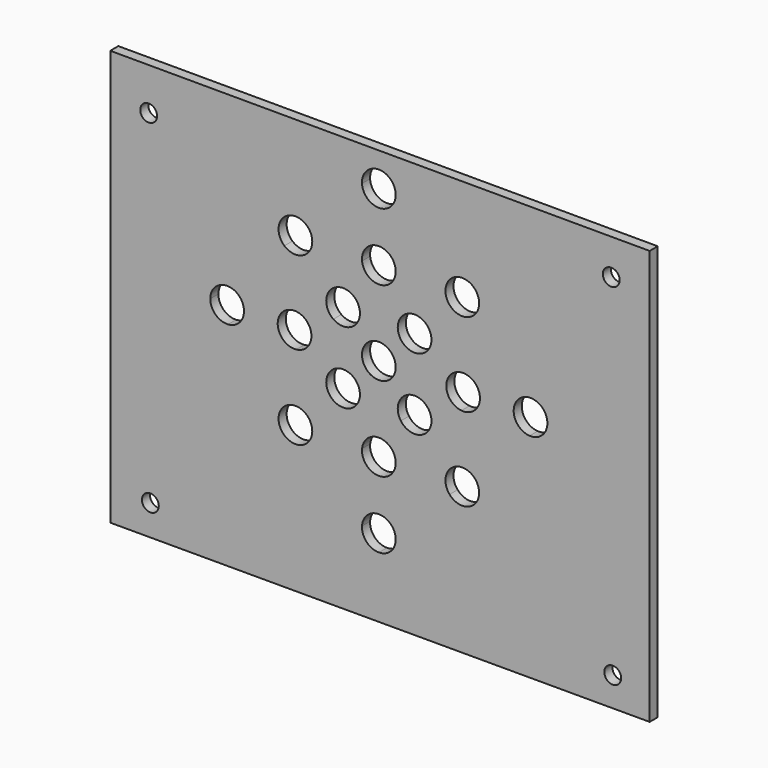
from build123d import *

# Parameters (mm, degrees)
F0_R     = 2.5
F0_R_2   = 5
F1_DEPTH = 3


with BuildPart() as f1:
    # F0 (on Front) → F1 (new body)
    with BuildSketch(Plane.XZ):
        Polygon((0, -68), (80, -68), (80, 55), (-80, 55.240198642), (-80, -68), align=None)
        with Locations((-68.1081116199, -58.9685998857)):
            Circle(F0_R, mode=Mode.SUBTRACT)
        with Locations((69.0506994724, -59.3423657119)):
            Circle(F0_R, mode=Mode.SUBTRACT)
        Polygon((49.6701618657, 0.1303526806), (49.6701618657, -49.8696473194), (-0.3298381532, -49.8696473194), (-50.3298381343, -49.8696473194), (-50.3298381343, 0.130352625), (-50.3298381343, 50.1303526806), (-0.3298380849, 50.1303526806), (49.6701618657, 50.1303526806), align=None, mode=Mode.SUBTRACT)
        with Locations((-68.6089098454, 42.6927655935)):
            Circle(F0_R, mode=Mode.SUBTRACT)
        with Locations((68.6089023948, 44.4455519319)):
            Circle(F0_R, mode=Mode.SUBTRACT)
        with BuildLine():
            ThreePointArc((-45.0520603566, -4.8619253071), (-32.1496432877, -31.6894524728), (-5.322116122, -44.5918695417))
            ThreePointArc((-5.322116122, -44.5918695417), (-0.3298381343, -39.8696473194), (4.6624398533, -44.5918695417))
            ThreePointArc((4.6624398533, -44.5918695417), (31.489967019, -31.6894524728), (44.3923840879, -4.8619253071))
            ThreePointArc((44.3923840879, -4.8619253071), (39.6701618657, 0.1303526806), (44.3923840879, 5.1226306682))
            ThreePointArc((44.3923840879, 5.1226306682), (31.489967019, 31.950157834), (4.6624398533, 44.8525749028))
            ThreePointArc((4.6624398533, 44.8525749028), (-0.3298381343, 40.1303526806), (-5.322116122, 44.8525749028))
            ThreePointArc((-5.322116122, 44.8525749028), (-32.1496432877, 31.950157834), (-45.0520603566, 5.1226306682))
            ThreePointArc((-45.0520603566, 5.1226306682), (-41.6974223481, 3.5662740353), (-40.3298381343, 0.1303526806))
            ThreePointArc((-40.3298381343, 0.1303526806), (-41.6974223481, -3.3055686741), (-45.0520603566, -4.8619253071))
        make_face()
        with BuildLine():
            ThreePointArc((27.6928642243, 21.1000487327), (32.8800593553, 11.1803621251), (34.6701618657, 0.1303526806))
            ThreePointArc((34.6701618657, 0.1303526806), (32.8800593553, -10.9196567639), (27.6928642243, -20.8393433716))
            ThreePointArc((27.6928642243, -20.8393433716), (28.9669661089, -22.5411058021), (29.4188992072, -24.618384661))
            ThreePointArc((29.4188992072, -24.618384661), (26.1660101872, -29.303211576), (20.6398579178, -27.8923496781))
            ThreePointArc((20.6398579178, -27.8923496781), (-0.3298381343, -34.8696473194), (-21.2995341865, -27.8923496781))
            ThreePointArc((-21.2995341865, -27.8923496781), (-28.6141093818, -28.1539185669), (-28.352540493, -20.8393433716))
            ThreePointArc((-28.352540493, -20.8393433716), (-35.3298381343, 0.1303526806), (-28.352540493, 21.1000487327))
            ThreePointArc((-28.352540493, 21.1000487327), (-28.6141093818, 28.414623928), (-21.2995341865, 28.1530550392))
            ThreePointArc((-21.2995341865, 28.1530550392), (-0.3298381343, 35.1303526806), (20.6398579178, 28.1530550392))
            ThreePointArc((20.6398579178, 28.1530550392), (26.1660101872, 29.5639169371), (29.4188992072, 24.8790900221))
            ThreePointArc((29.4188992072, 24.8790900221), (28.9669661089, 22.8018111633), (27.6928642243, 21.1000487327))
        make_face(mode=Mode.SUBTRACT)
        with BuildLine():
            ThreePointArc((27.6928642243, -20.8393433716), (32.8800593553, -10.9196567639), (34.6701618657, 0.1303526806))
            ThreePointArc((34.6701618657, 0.1303526806), (32.8800593553, 11.1803621251), (27.6928642243, 21.1000487327))
            ThreePointArc((27.6928642243, 21.1000487327), (20.8833653012, 21.3435561162), (20.6398579178, 28.1530550392))
            ThreePointArc((20.6398579178, 28.1530550392), (-0.3298381343, 35.1303526806), (-21.2995341865, 28.1530550392))
            ThreePointArc((-21.2995341865, 28.1530550392), (-20.3937485609, 26.6262010021), (-20.0785754759, 24.8790900221))
            ThreePointArc((-20.0785754759, 24.8790900221), (-23.0012966171, 20.3310231204), (-28.352540493, 21.1000487327))
            ThreePointArc((-28.352540493, 21.1000487327), (-35.3298381343, 0.1303526806), (-28.352540493, -20.8393433716))
            ThreePointArc((-28.352540493, -20.8393433716), (-23.0012966171, -20.0703177592), (-20.0785754759, -24.618384661))
            ThreePointArc((-20.0785754759, -24.618384661), (-20.3937485609, -26.365495641), (-21.2995341865, -27.8923496781))
            ThreePointArc((-21.2995341865, -27.8923496781), (-0.3298381343, -34.8696473194), (20.6398579178, -27.8923496781))
            ThreePointArc((20.6398579178, -27.8923496781), (20.8833653012, -21.082850755), (27.6928642243, -20.8393433716))
        make_face()
        with BuildLine():
            ThreePointArc((4.6450990512, 24.6303526806), (17.3478313953, 17.8080222102), (24.1701618657, 5.1052898661))
            ThreePointArc((24.1701618657, 5.1052898661), (28.0242638319, 3.8384519241), (29.6701618657, 0.1303526806))
            ThreePointArc((29.6701618657, 0.1303526806), (28.0242638319, -3.577746563), (24.1701618657, -4.844584505))
            ThreePointArc((24.1701618657, -4.844584505), (17.3478313953, -17.5473168491), (4.6450990512, -24.3696473194))
            ThreePointArc((4.6450990512, -24.3696473194), (4.6638922312, -24.6193334441), (4.6701618657, -24.8696473194))
            ThreePointArc((4.6701618657, -24.8696473194), (-0.5801520096, -29.863377685), (-5.3047753199, -24.3696473194))
            ThreePointArc((-5.3047753199, -24.3696473194), (-18.007507664, -17.5473168491), (-24.8298381343, -4.844584505))
            ThreePointArc((-24.8298381343, -4.844584505), (-30.3298381343, 0.1303526806), (-24.8298381343, 5.1052898661))
            ThreePointArc((-24.8298381343, 5.1052898661), (-18.007507664, 17.8080222102), (-5.3047753199, 24.6303526806))
            ThreePointArc((-5.3047753199, 24.6303526806), (-0.5801520096, 30.1240830461), (4.6701618657, 25.1303526806))
            ThreePointArc((4.6701618657, 25.1303526806), (4.6638922312, 24.8800388053), (4.6450990512, 24.6303526806))
        make_face(mode=Mode.SUBTRACT)
        with BuildLine():
            ThreePointArc((24.1701618657, -4.844584505), (19.6701618657, 0.1303526806), (24.1701618657, 5.1052898661))
            ThreePointArc((24.1701618657, 5.1052898661), (17.3478313953, 17.8080222102), (4.6450990512, 24.6303526806))
            ThreePointArc((4.6450990512, 24.6303526806), (-0.3298381343, 20.1303526806), (-5.3047753199, 24.6303526806))
            ThreePointArc((-5.3047753199, 24.6303526806), (-18.007507664, 17.8080222102), (-24.8298381343, 5.1052898661))
            ThreePointArc((-24.8298381343, 5.1052898661), (-21.6217388908, 3.4844546468), (-20.3298381343, 0.1303526806))
            ThreePointArc((-20.3298381343, 0.1303526806), (-21.6217388908, -3.2237492857), (-24.8298381343, -4.844584505))
            ThreePointArc((-24.8298381343, -4.844584505), (-18.007507664, -17.5473168491), (-5.3047753199, -24.3696473194))
            ThreePointArc((-5.3047753199, -24.3696473194), (-0.3298381343, -19.8696473194), (4.6450990512, -24.3696473194))
            ThreePointArc((4.6450990512, -24.3696473194), (17.3478313953, -17.5473168491), (24.1701618657, -4.844584505))
        make_face()
        with BuildLine():
            ThreePointArc((13.1735913764, 6.6616153035), (14.2912330073, 3.4806181431), (14.6701618657, 0.1303526806))
            ThreePointArc((14.6701618657, 0.1303526806), (14.2912330073, -3.219912782), (13.1735913764, -6.4009099423))
            ThreePointArc((13.1735913764, -6.4009099423), (14.7199684496, -8.1832312619), (15.2767635834, -10.4762490372))
            ThreePointArc((15.2767635834, -10.4762490372), (11.7971754562, -15.2394777465), (6.2014244886, -13.3730768301))
            ThreePointArc((6.2014244886, -13.3730768301), (-0.3298381343, -14.8696473194), (-6.8611007573, -13.3730768301))
            ThreePointArc((-6.8611007573, -13.3730768301), (-14.4719737581, -14.0117829432), (-13.833267645, -6.4009099423))
            ThreePointArc((-13.833267645, -6.4009099423), (-15.3298381343, 0.1303526806), (-13.833267645, 6.6616153035))
            ThreePointArc((-13.833267645, 6.6616153035), (-14.4719737581, 14.2724883043), (-6.8611007573, 13.6337821913))
            ThreePointArc((-6.8611007573, 13.6337821913), (-0.3298381343, 15.1303526806), (6.2014244886, 13.6337821913))
            ThreePointArc((6.2014244886, 13.6337821913), (11.7971754562, 15.5001831077), (15.2767635834, 10.7369543984))
            ThreePointArc((15.2767635834, 10.7369543984), (14.7199684496, 8.4439366231), (13.1735913764, 6.6616153035))
        make_face(mode=Mode.SUBTRACT)
        with BuildLine():
            Line((-0.3298381532, -49.8696473194), (49.6701618657, -49.8696473194))
            Line((49.6701618657, -49.8696473194), (49.6701618657, 0.1303526806))
            ThreePointArc((49.6701618657, 0.1303526806), (48.1060832203, -3.5020631057), (44.3923840879, -4.8619253071))
            ThreePointArc((44.3923840879, -4.8619253071), (31.489967019, -31.6894524728), (4.6624398533, -44.5918695417))
            ThreePointArc((4.6624398533, -44.5918695417), (4.6682309897, -44.7307047744), (4.6701618657, -44.8696473194))
            ThreePointArc((4.6701618657, -44.8696473194), (3.2056957649, -48.405181232), (-0.3298381532, -49.8696473194))
        make_face()
        with BuildLine():
            Line((-50.3298381343, -49.8696473194), (-0.3298381532, -49.8696473194))
            ThreePointArc((-0.3298381532, -49.8696473194), (-3.9622539271, -48.3055686673), (-5.322116122, -44.5918695417))
            ThreePointArc((-5.322116122, -44.5918695417), (-32.1496432877, -31.6894524728), (-45.0520603566, -4.8619253071))
            ThreePointArc((-45.0520603566, -4.8619253071), (-48.7657594688, -3.5020631248), (-50.3298381343, 0.130352625))
            Line((-50.3298381343, 0.130352625), (-50.3298381343, -49.8696473194))
        make_face()
        with BuildLine():
            ThreePointArc((44.3923840879, 5.1226306682), (48.1060832203, 3.7627684669), (49.6701618657, 0.1303526806))
            Line((49.6701618657, 0.1303526806), (49.6701618657, 50.1303526806))
            Line((49.6701618657, 50.1303526806), (-0.3298380849, 50.1303526806))
            ThreePointArc((-0.3298380849, 50.1303526806), (3.205695789, 48.665886569), (4.6701618657, 45.1303526806))
            ThreePointArc((4.6701618657, 45.1303526806), (4.6682309897, 44.9914101355), (4.6624398533, 44.8525749028))
            ThreePointArc((4.6624398533, 44.8525749028), (31.489967019, 31.950157834), (44.3923840879, 5.1226306682))
        make_face()
        with BuildLine():
            Line((-50.3298381343, 50.1303526806), (-50.3298381343, 0.130352625))
            ThreePointArc((-50.3298381343, 0.130352625), (-48.7657595092, 3.7627684478), (-45.0520603566, 5.1226306682))
            ThreePointArc((-45.0520603566, 5.1226306682), (-32.1496432877, 31.950157834), (-5.322116122, 44.8525749028))
            ThreePointArc((-5.322116122, 44.8525749028), (-3.9622539037, 48.5662740532), (-0.3298380849, 50.1303526806))
            Line((-0.3298380849, 50.1303526806), (-50.3298381343, 50.1303526806))
        make_face()
        with BuildLine():
            ThreePointArc((13.1735913764, -6.4009099423), (14.2912330073, -3.219912782), (14.6701618657, 0.1303526806))
            ThreePointArc((14.6701618657, 0.1303526806), (14.2912330073, 3.4806181431), (13.1735913764, 6.6616153035))
            ThreePointArc((13.1735913764, 6.6616153035), (6.7412296775, 7.2014204924), (6.2014244886, 13.6337821913))
            ThreePointArc((6.2014244886, 13.6337821913), (-0.3298381343, 15.1303526806), (-6.8611007573, 13.6337821913))
            ThreePointArc((-6.8611007573, 13.6337821913), (-6.1732111428, 12.2573662711), (-5.9364398521, 10.7369543984))
            ThreePointArc((-5.9364398521, 10.7369543984), (-8.6434220769, 6.2937495323), (-13.833267645, 6.6616153035))
            ThreePointArc((-13.833267645, 6.6616153035), (-15.3298381343, 0.1303526806), (-13.833267645, -6.4009099423))
            ThreePointArc((-13.833267645, -6.4009099423), (-8.6434220769, -6.0330441711), (-5.9364398521, -10.4762490372))
            ThreePointArc((-5.9364398521, -10.4762490372), (-6.1732111428, -11.99666091), (-6.8611007573, -13.3730768301))
            ThreePointArc((-6.8611007573, -13.3730768301), (-0.3298381343, -14.8696473194), (6.2014244886, -13.3730768301))
            ThreePointArc((6.2014244886, -13.3730768301), (6.7412296775, -6.9407151313), (13.1735913764, -6.4009099423))
        make_face()
        with Locations((-0.3298381343, 0.1303526806)):
            Circle(F0_R_2, mode=Mode.SUBTRACT)
    extrude(amount=F1_DEPTH)


solid = f1.part
